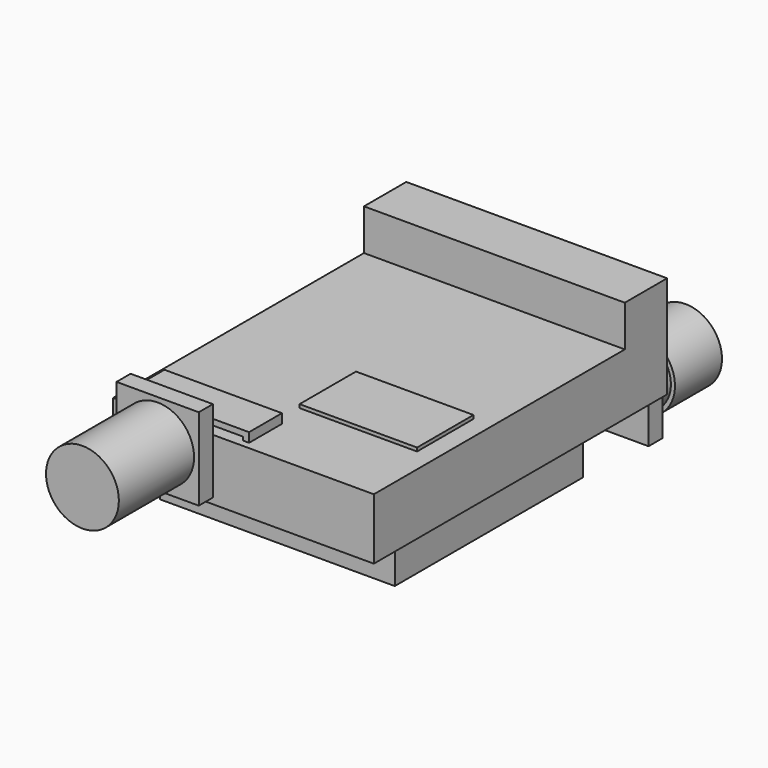
from build123d import *

# Parameters (mm, degrees)
F0_W      = 22
F0_H      = 30
F1_DEPTH  = 1.5
F2_W      = 6.5
F2_H      = 6.5
F3_DEPTH  = 1.5
F4_R      = 2.75
F5_DEPTH  = 1.5
F6_R      = 3.1
F7_DEPTH  = 5
F8_W      = 20
F8_H      = 20
F9_DEPTH  = 3.5
F10_W     = 10
F10_H     = 3.5
F11_DEPTH = 4.5
F12_W     = 9
F12_H     = 2
F13_DEPTH = 3
F12_H_2   = 1
F14_DEPTH = 25
F15_W     = 10
F15_H     = 6
F16_DEPTH = 4
F17_W     = 22.2
F17_H     = 31.2
F18_DEPTH = 8.7
F19_R     = 3.1
F20_DEPTH = 9.5
F21_W     = 22.2
F21_H     = 26.7
F22_DEPTH = 3.5
F23_W     = 7
F23_H     = 7
F24_DEPTH = 1.5


with BuildPart() as f1:
    # F0 (on Top) → F1 (new body)
    with BuildSketch(Plane.XY):
        Rectangle(F0_W, F0_H)
    extrude(amount=F1_DEPTH)

    # F2 (on face) → F3 (join)
    with BuildSketch(Plane(origin=(0, 15, 0), x_dir=(-1, 0, 0), z_dir=(0, 1, 0))):
        with Locations((-6.75, -0.75)):
            Rectangle(F2_W, F2_H)
    extrude(amount=F3_DEPTH)

    # F4 (on face) → F5 (join)
    with BuildSketch(Plane(origin=(0, 16.5, 0), x_dir=(-1, 0, 0), z_dir=(0, 1, 0))):
        with Locations((-6.75, -0.75)):
            Circle(F4_R)
    extrude(amount=F5_DEPTH)

    # F6 (on face) → F7 (join)
    with BuildSketch(Plane(origin=(0, 18, 0), x_dir=(-1, 0, 0), z_dir=(0, 1, 0))):
        with Locations((-6.75, -0.75)):
            Circle(F6_R)
    extrude(amount=F7_DEPTH)

    # F8 (on face) → F9 (join)
    with BuildSketch(Plane(origin=(0, 0, 0), x_dir=(1, 0, 0), z_dir=(0, 0, -1))):
        with Locations((0, 2)):
            Rectangle(F8_W, F8_H)
    extrude(amount=F9_DEPTH)

    # F10 (on face) → F11 (join)
    with BuildSketch(Plane.XY.offset(1.5)):
        with Locations((-5, -13.25)):
            Rectangle(F10_W, F10_H)
    extrude(amount=F11_DEPTH)

    # F12 (on face) → F13 (cut)
    with BuildSketch(Plane.XZ.offset(15)):
        with Locations((-5, 3)):
            Rectangle(F12_W, F12_H)
    extrude(amount=-F13_DEPTH, mode=Mode.SUBTRACT)

    # F12 (on face) → F14 (cut)
    with BuildSketch(Plane.XZ.offset(15)):
        with Locations((-5, 5)):
            Rectangle(F12_W, F12_H_2)
    extrude(amount=-F14_DEPTH, mode=Mode.SUBTRACT)

    # F15 (on face) → F16 (join)
    with BuildSketch(Plane.XY.offset(1.5)):
        with Locations((4.5, -6)):
            Rectangle(F15_W, F15_H)
    extrude(amount=F16_DEPTH)


with BuildPart() as f18:
    # F17 (on Top) → F18 (new body)
    with BuildSketch(Plane.XY):
        Rectangle(F17_W, F17_H)
    extrude(amount=F18_DEPTH)

    # F19 (on face) → F20 (join)
    with BuildSketch(Plane.XZ.offset(15.6)):
        with Locations((-6.1, 4)):
            Circle(F19_R)
    extrude(amount=F20_DEPTH)

    # F21 (on face) → F22 (cut)
    with BuildSketch(Plane.XY.offset(8.7)):
        with Locations((0, -2.25)):
            Rectangle(F21_W, F21_H)
    extrude(amount=-F22_DEPTH, mode=Mode.SUBTRACT)

    # F23 (on face) → F24 (join)
    with BuildSketch(Plane.XZ.offset(15.6)):
        with Locations((-6.1, 4)):
            Rectangle(F23_W, F23_H)
    extrude(amount=F24_DEPTH)


solid = Compound([f1.part, f18.part])
